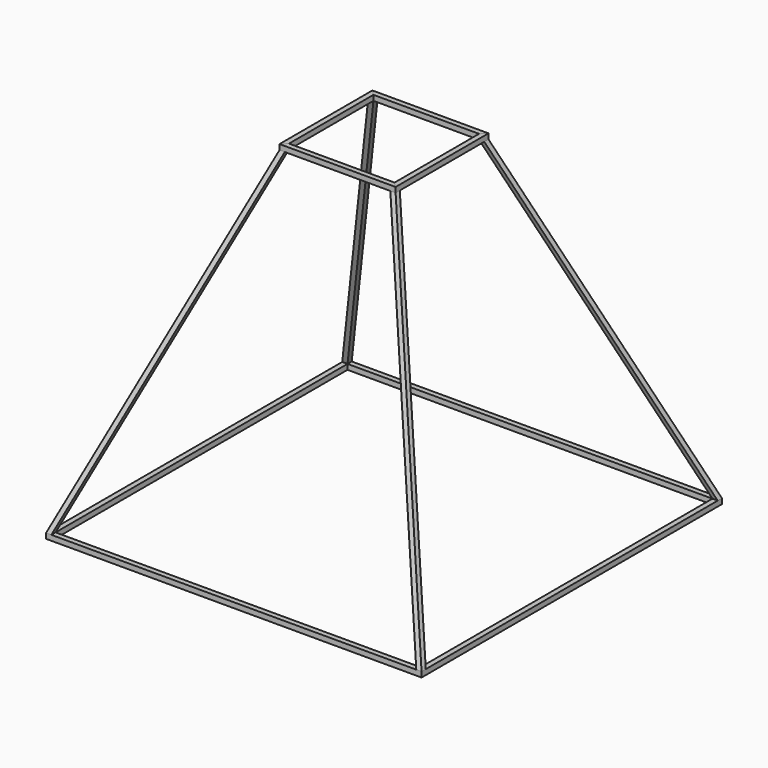
from build123d import *

# Parameters (mm, degrees)
F0_W      = 3.175
F0_H      = 3.175
F1_DEPTH  = 226.35
F2_SIZE   = 3.17499
F2_2_SIZE = 3.17499
F5_ANGLE  = 90
F8_DEPTH  = 3.175
F9_SIZE   = 3.17499
F9_2_SIZE = 3.17499
F10_ANGLE = 90
F12_W     = 3.175
F12_H     = 3.175
F20_ANGLE = 90
F21_ANGLE = 180


# Not quite as in the source:
# - a fillet or chamfer is up to 0.001 mm smaller than in the source, because OpenCascade refuses the exact size


with BuildPart() as f1:
    # F0 (on Front) → F1 (new body)
    with BuildSketch(Plane.XZ):
        with Locations((1.5875, 1.5875)):
            Rectangle(F0_W, F0_H)
    extrude(amount=F1_DEPTH)

    # F2 (size 3.175 in the source; OpenCascade refuses exactly that, so slightly less here)
    f2_edges = [f1.edges().sort_by_distance(p)[0] for p in [
        (3.175, -226.35, 1.5875),
        (3.175, 0, 1.5875),
    ]]
    chamfer(f2_edges, length=F2_SIZE)


with BuildPart() as f1b:
    # F0 (on Front) → F1, piece 2 (new body)
    with BuildSketch(Plane.XZ):
        with Locations((224.7625, 1.5875)):
            Rectangle(F0_W, F0_H)
    extrude(amount=F1_DEPTH)

    # F2#2 (size 3.175 in the source; OpenCascade refuses exactly that, so slightly less here)
    f2_2_edges = [f1b.edges().sort_by_distance(p)[0] for p in [
        (223.175, -226.35, 1.5875),
        (223.175, 0, 1.5875),
    ]]
    chamfer(f2_2_edges, length=F2_2_SIZE)


with BuildPart() as f5_1:
    # F5: copy of F1
    add(f1.part.rotate(Axis((113.175, -113.175, 5), (0, 0, -1)), F5_ANGLE))


with BuildPart() as f5_2:
    # F5: copy of F1b
    add(f1b.part.rotate(Axis((113.175, -113.175, 5), (0, 0, -1)), F5_ANGLE))


with BuildPart() as f8:
    # F7 (on offset) → F8 (new body)
    with BuildSketch(Plane.XY.offset(200)):
        Polygon((81.35, -148.175), (81.35, -113.175), (81.35, -78.175), (78.175, -78.175), (78.175, -113.175), (78.175, -148.175), align=None)
    extrude(amount=F8_DEPTH)

    # F9 (size 3.175 in the source; OpenCascade refuses exactly that, so slightly less here)
    f9_edges = [f8.edges().sort_by_distance(p)[0] for p in [
        (81.35, -148.175, 201.5875),
        (81.35, -78.175, 201.5875),
    ]]
    chamfer(f9_edges, length=F9_SIZE)


with BuildPart() as f8b:
    # F7 (on offset) → F8, piece 2 (new body)
    with BuildSketch(Plane.XY.offset(200)):
        Polygon((148.175, -78.175), (145, -78.175), (145, -113.175), (145, -148.175), (148.175, -148.175), (148.175, -113.175), align=None)
    extrude(amount=F8_DEPTH)

    # F9#2 (size 3.175 in the source; OpenCascade refuses exactly that, so slightly less here)
    f9_2_edges = [f8b.edges().sort_by_distance(p)[0] for p in [
        (145, -148.175, 201.5875),
        (145, -78.175, 201.5875),
    ]]
    chamfer(f9_2_edges, length=F9_2_SIZE)


with BuildPart() as f10_1:
    # F10: copy of F8
    add(f8.part.rotate(Axis((113.175, -113.175, 5), (0, 0, -1)), F10_ANGLE))


with BuildPart() as f10_2:
    # F10: copy of F8b
    add(f8b.part.rotate(Axis((113.175, -113.175, 5), (0, 0, -1)), F10_ANGLE))


with BuildPart() as f19:
    # F19: sweep along a path in F18
    with BuildLine(Plane(origin=(0, 0, 0), x_dir=(0.7071067812, -0.7071067812, 0), z_dir=(-0.7071067812, -0.7071067812, 0))) as f19_path:
        Line((2.2450640303, 3.175), (112.8012092688, 200))
    # F12 (on offset) → F19 (sweep)
    with BuildSketch(Plane.XY.offset(200)):
        with Locations((79.7625, -79.7625)):
            Rectangle(F12_W, F12_H)
    sweep(path=f19_path.line)


with BuildPart() as f20_1:
    # F20: copy of F19
    add(f19.part.rotate(Axis((113.175, -113.175, 5), (0, 0, -1)), F20_ANGLE))


with BuildPart() as f21_1:
    # F21: copy of F19
    add(f19.part.rotate(Axis((113.175, -113.175, 5), (0, 0, -1)), F21_ANGLE))


with BuildPart() as f21_2:
    # F21: copy of F20_1
    add(f20_1.part.rotate(Axis((113.175, -113.175, 5), (0, 0, -1)), F21_ANGLE))


solid = Compound([f1.part, f1b.part, f5_1.part, f5_2.part, f8.part, f8b.part, f10_1.part, f10_2.part, f19.part, f20_1.part, f21_1.part, f21_2.part])
